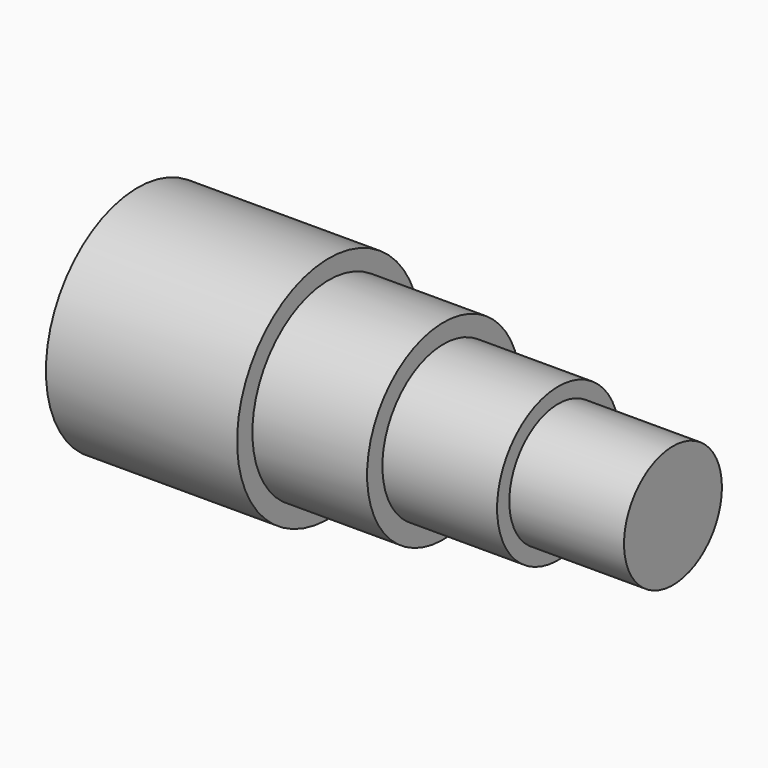
from build123d import *

# Parameters (mm, degrees)
F0_R     = 15
F1_DEPTH = 25
F2_R     = 12.5
F3_DEPTH = 15
F4_R     = 10
F5_DEPTH = 15
F6_R     = 8
F7_DEPTH = 15


# Not quite as in the source:
# - the program builds the solid bodies; features that only make, move or delete a surface that nothing else refers to are left out


with BuildPart() as f1:
    # F0 (on Right) → F1 (new body)
    with BuildSketch(Plane.YZ):
        Circle(F0_R)
    extrude(amount=-F1_DEPTH)

    # F2 (on face) → F3 (join)
    with BuildSketch(Plane.YZ):
        Circle(F2_R)
    extrude(amount=F3_DEPTH)

    # F4 (on face) → F5 (join)
    with BuildSketch(Plane.YZ.offset(15)):
        Circle(F4_R)
    extrude(amount=F5_DEPTH)

    # F6 (on face) → F7 (join)
    with BuildSketch(Plane.YZ.offset(30)):
        Circle(F6_R)
    extrude(amount=F7_DEPTH)


solid = f1.part
